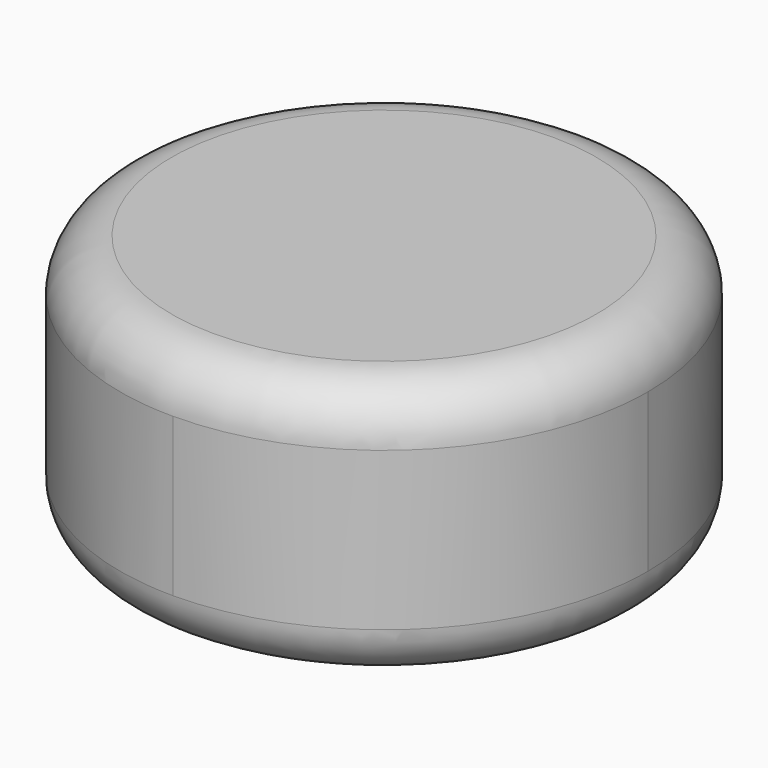
from build123d import *

# Parameters (mm, degrees)
F1_DEPTH = 25.4


# Not quite as in the source:
# - a fillet or chamfer that OpenCascade refuses, or shapes differently, is made with other operations: its cross-section is extruded or revolved along the edge and cut away or added


with BuildPart() as f1:
    # F0 (on Top) → F1 (new body)
    with BuildSketch(Plane.XY):
        with BuildLine():
            Line((0, 0), (25.6860326238, 0))
            ThreePointArc((25.6860326238, 0), (18.1627678501, 18.1627678501), (0, 25.6860326238))
            Line((0, 25.6860326238), (0, 0))
        make_face()
        with BuildLine():
            ThreePointArc((0, -25.6860326238), (18.1627678501, -18.1627678501), (25.6860326238, 0))
            Line((25.6860326238, 0), (0, 0))
            Line((0, 0), (0, -25.6860326238))
        make_face()
        with BuildLine():
            ThreePointArc((-25.6860326238, 0), (-18.1627678501, -18.1627678501), (0, -25.6860326238))
            Line((0, -25.6860326238), (0, 0))
            Line((0, 0), (-25.6860326238, 0))
        make_face()
        with BuildLine():
            Line((0, 0), (0, 25.6860326238))
            ThreePointArc((0, 25.6860326238), (-18.1627678501, 18.1627678501), (-25.6860326238, 0))
            Line((-25.6860326238, 0), (0, 0))
        make_face()
    extrude(amount=F1_DEPTH)

    # F2: fillet of radius 5.08 on 3 edges, made by hand

    # F2_s1 → F2_t2 (revolve, cut)
    with BuildSketch(Plane.YZ):
        with BuildLine():
            ThreePointArc((25.6864326238, 20.3190343146), (24.1981350723, 23.9121024484), (20.6050669384, 25.4004))
            Line((20.6050669384, 25.4004), (20.6050669384, 25.9085365685))
            ThreePointArc((20.6050669384, 25.9085365685), (23.1455497811, 25.9081365685), (25.6860326238, 25.9081365685))
            Line((25.6860326238, 25.9081365685), (26.1941691924, 25.4))
            ThreePointArc((26.1941691924, 25.4), (26.1941691924, 22.8595171573), (26.1945691924, 20.3190343146))
            Line((26.1945691924, 20.3190343146), (25.6864326238, 20.3190343146))
        make_face()
    revolve(axis=Axis((0, 0, 25.4), (0, 0, 1)), mode=Mode.SUBTRACT)

    # F2_s3 → F2_t4 (revolve, cut)
    with BuildSketch(Plane.YZ):
        with BuildLine():
            ThreePointArc((25.6864326238, 5.0809656854), (24.1981350723, 1.4878975516), (20.6050669384, -0.0004))
            Line((20.6050669384, -0.0004), (20.6050669384, -0.5085365685))
            ThreePointArc((20.6050669384, -0.5085365685), (23.1455497811, -0.5081365685), (25.6860326238, -0.5081365685))
            Line((25.6860326238, -0.5081365685), (26.1941691924, 0))
            ThreePointArc((26.1941691924, 0), (26.1941691924, 2.5404828427), (26.1945691924, 5.0809656854))
            Line((26.1945691924, 5.0809656854), (25.6864326238, 5.0809656854))
        make_face()
    revolve(axis=Axis((0, 0, 0), (0, 0, 1)), mode=Mode.SUBTRACT)


solid = f1.part
